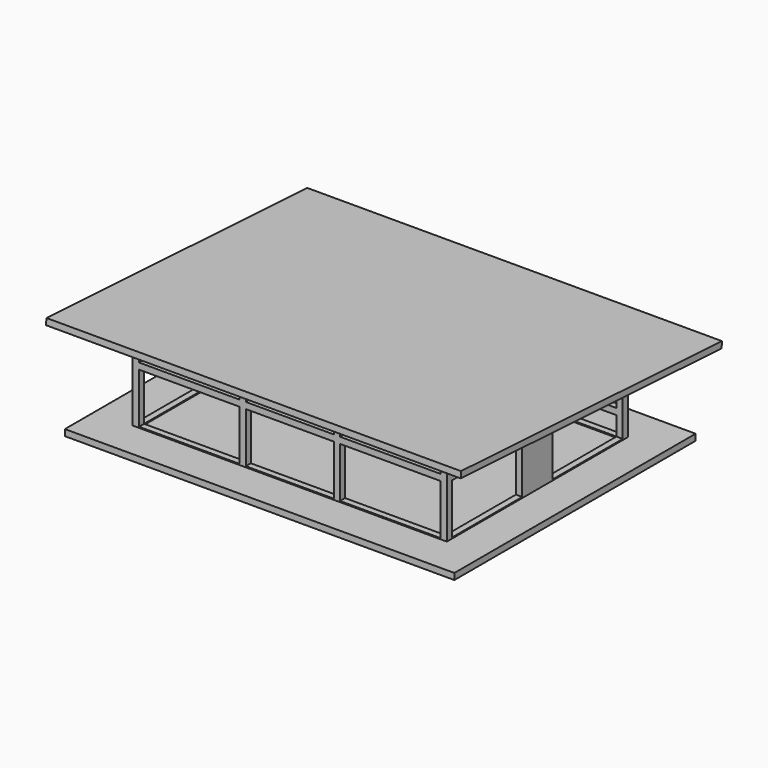
from build123d import *

# Parameters (mm, degrees)
F0_W      = 18897.6
F0_H      = 14630.4
F1_DEPTH  = 304.8
F2_W      = 15240
F2_H      = 10972.8
F3_DEPTH  = 4267.2
F5_DEPTH  = 15240
F6_T      = -304.8
F7_W      = 20116.8
F7_H      = 15849.6
F7_W_2    = 15240
F7_H_2    = 10989.7202876142
F7_W_3    = 14630.4
F7_H_3    = 10379.1802716357
F8_DEPTH  = 304.8
F9_W      = 4267.2
F9_H      = 2438.4
F9_W_2    = 4876.8
F10_DEPTH = 10972.8
F11_W     = 4267.2
F11_H     = 2438.4
F12_DEPTH = 15240
F13_W     = 4876.8
F13_H     = 1168.4
F13_W_2   = 4267.2
F14_DEPTH = 304.8
F16_DEPTH = 15240
F18_W     = 4876.8
F18_H     = 304.8000000003
F18_W_2   = 4267.2
F19_DEPTH = 304.8


with BuildPart() as f1:
    # F0 (on Top) → F1 (new body)
    with BuildSketch(Plane.XY):
        Rectangle(F0_W, F0_H)
    extrude(amount=-F1_DEPTH)


with BuildPart() as f3:
    # F2 (on face) → F3 (new body)
    with BuildSketch(Plane.XY):
        Rectangle(F2_W, F2_H)
    extrude(amount=F3_DEPTH)

    # F4 (on face) → F5 (cut, through all)
    with BuildSketch(Plane(origin=(-7620, 0, 0), x_dir=(0, -1, 0), z_dir=(-1, 0, 0))):
        Polygon((-5486.4, 4267.2), (-5486.4, 3657.6), (5486.4, 4267.2), align=None)
    extrude(amount=-F5_DEPTH, mode=Mode.SUBTRACT)

    # F6
    f6_openings = [f3.faces().sort_by_distance(p)[0] for p in [
        (0, 0, 3962.4),
        (0, 0, 0),
    ]]
    offset(amount=F6_T, openings=f6_openings)

    # F9 (on face) → F10 (cut, through all)
    with BuildSketch(Plane.XZ.offset(5486.4)):
        with Locations((0, 1270)):
            Rectangle(F9_W, F9_H)
        with Locations((4876.8, 1270)):
            Rectangle(F9_W_2, F9_H)
        with Locations((-4876.8, 1270)):
            Rectangle(F9_W_2, F9_H)
    extrude(amount=-F10_DEPTH, mode=Mode.SUBTRACT)

    # F11 (on face) → F12 (cut, through all)
    with BuildSketch(Plane(origin=(-7620, 0, 0), x_dir=(0, -1, 0), z_dir=(-1, 0, 0))):
        with Locations((-3048, 1270)):
            Rectangle(F11_W, F11_H)
        with Locations((3048, 1270)):
            Rectangle(F11_W, F11_H)
    extrude(amount=-F12_DEPTH, mode=Mode.SUBTRACT)

    # F13 (on face) → F14 (cut, through all)
    with BuildSketch(Plane.XZ.offset(5486.4)):
        with Locations((4876.8, 3378.2)):
            Rectangle(F13_W, F13_H)
        with Locations((0, 3378.2)):
            Rectangle(F13_W_2, F13_H)
        with Locations((-4876.8, 3378.2)):
            Rectangle(F13_W, F13_H)
    extrude(amount=-F14_DEPTH, mode=Mode.SUBTRACT)

    # F15 (on face) → F16 (cut, through all)
    with BuildSketch(Plane(origin=(-7620, 0, 0), x_dir=(0, -1, 0), z_dir=(-1, 0, 0))):
        Polygon((-5181.6, 2794), (-914.4, 2794), (-914.4, 3606.3299920107), (-5181.6, 3369.263325344), align=None)
        Polygon((914.4, 2794), (5181.6, 2794), (5181.6, 3944.9966586774), (914.4, 3707.9299920107), align=None)
    extrude(amount=-F16_DEPTH, mode=Mode.SUBTRACT)

    # F18 (on offset) → F19 (join)
    with BuildSketch(Plane.XY.offset(965.2)):
        with Locations((4876.8, 5334.0000000002)):
            Rectangle(F18_W, F18_H)
        with Locations((0, 5334.0000000002)):
            Rectangle(F18_W_2, F18_H)
        with Locations((-4876.8, 5334.0000000002)):
            Rectangle(F18_W, F18_H)
    extrude(amount=F19_DEPTH)


with BuildPart() as f8:
    # F7 (on face) → F8 (new body)
    with BuildSketch(Plane(origin=(0, 219.456, 3950.208), x_dir=(1, 0, 0), z_dir=(0, 0.0554700196, 0.9984603532))):
        Rectangle(F7_W, F7_H)
        with Locations((0, -219.7944057523)):
            Rectangle(F7_W_2, F7_H_2, mode=Mode.SUBTRACT)
        with Locations((0, -219.7944057523)):
            Rectangle(F7_W_2, F7_H_2)
        with Locations((0, -219.7944057523)):
            Rectangle(F7_W_3, F7_H_3, mode=Mode.SUBTRACT)
        with Locations((0, -219.7944057523)):
            Rectangle(F7_W_3, F7_H_3)
    extrude(amount=F8_DEPTH)


solid = Compound([f1.part, f3.part, f8.part])
